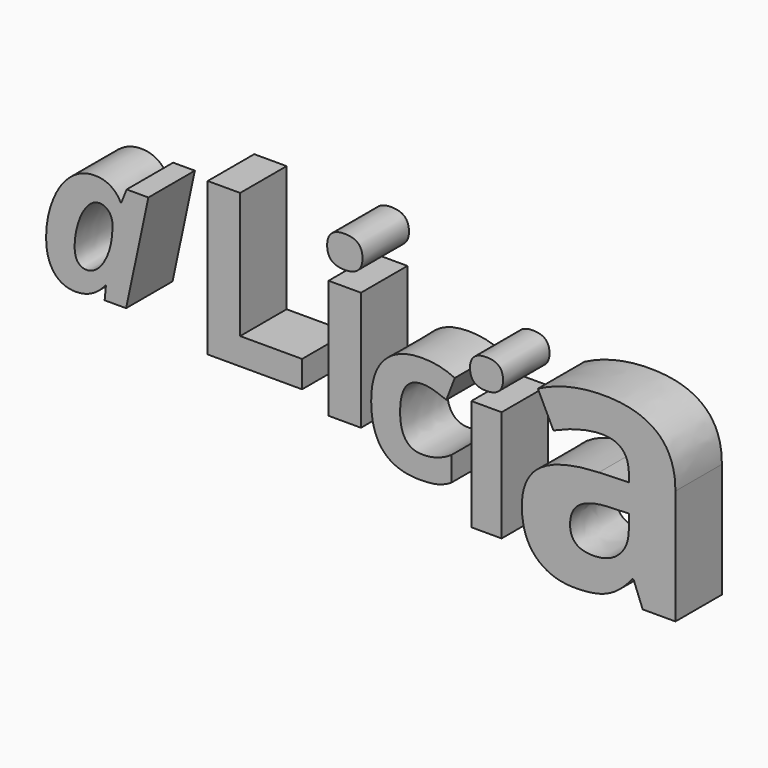
from build123d import *

# Parameters (mm, degrees)
F2_TEXT_SIZE = 95.2418427914
F3_DEPTH     = 25.4
F4_TEXT_SIZE = 83.4313790417
F5_DEPTH     = 25.4
F7_TEXT_SIZE = 137.9983137465
F8_DEPTH     = 25.4
F1_TEXT_SIZE = 93.5624043147
F9_DEPTH     = 25.4
F0_TEXT_SIZE = 83.9069201094
F10_DEPTH    = 25.4
F6_TEXT_SIZE = 89.0207806757
F11_DEPTH    = 25.4


# Not quite as in the source:
# - Text() gives the source's letters only with a copy of the font that has no kerning and outlines rounded to 1/6400 em; it was checked with that copy


with BuildPart() as f3:
    # F2 (on Front) → F3 (new body)
    with BuildSketch(Plane.XZ):
        with Locations((-97.6916328073, -49.2619387805)):
            Text('i', F2_TEXT_SIZE, font='Open Sans', font_style=FontStyle.BOLD, text_align=(TextAlign.LEFT, TextAlign.BOTTOM))
    extrude(amount=F3_DEPTH)


with BuildPart() as f5:
    # F4 (on Front) → F5 (new body)
    with BuildSketch(Plane.XZ):
        with Locations((-75.362123549, -60.0705929101)):
            Text('c', F4_TEXT_SIZE, font='Open Sans', font_style=FontStyle.BOLD, text_align=(TextAlign.LEFT, TextAlign.BOTTOM))
    extrude(amount=F5_DEPTH)


with BuildPart() as f8:
    # F7 (on Front) → F8 (new body)
    with BuildSketch(Plane.XZ):
        with Locations((-11.5170897916, -79.1119560599)):
            Text('a', F7_TEXT_SIZE, font='Open Sans', font_style=FontStyle.BOLD, text_align=(TextAlign.LEFT, TextAlign.BOTTOM))
    extrude(amount=F8_DEPTH)


with BuildPart() as f9:
    # F1 (on Front) → F9 (new body)
    with BuildSketch(Plane.XZ):
        with Locations((-151.4854729176, -42.8377538919)):
            Text('L', F1_TEXT_SIZE, font='Open Sans', font_style=FontStyle.BOLD, text_align=(TextAlign.LEFT, TextAlign.BOTTOM))
    extrude(amount=F9_DEPTH)


with BuildPart() as f10:
    # F0 (on Front) → F10 (new body)
    with BuildSketch(Plane.XZ):
        with Locations((-217.4590379, -36.6393327713)):
            Text('a', F0_TEXT_SIZE, font='Open Sans', font_style=FontStyle.BOLDITALIC, text_align=(TextAlign.LEFT, TextAlign.BOTTOM))
    extrude(amount=F10_DEPTH)


with BuildPart() as f11:
    # F6 (on Front) → F11 (new body)
    with BuildSketch(Plane.XZ):
        with Locations((-34.7741022706, -71.8714669347)):
            Text('i', F6_TEXT_SIZE, font='Open Sans', font_style=FontStyle.BOLD, text_align=(TextAlign.LEFT, TextAlign.BOTTOM))
    extrude(amount=F11_DEPTH)


solid = Compound([f3.part, f5.part, f8.part, f9.part, f10.part, f11.part])
